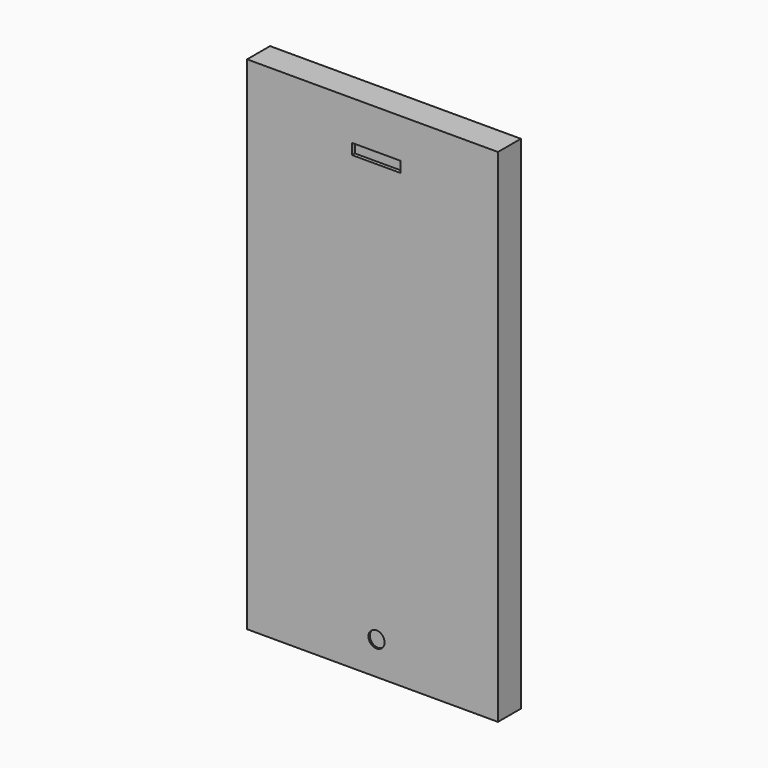
from build123d import *

# Parameters (mm, degrees)
F0_W     = 70
F0_H     = 140
F1_DEPTH = 8
F2_W     = 13.5
F2_H     = 3
F3_DEPTH = 1
F4_R     = 2.25
F5_DEPTH = 0.5
F6_R     = 5
F7_DEPTH = 1


# Not quite as in the source:
# - a feature of the source that left no trace in its solid (it failed there, or was rolled back) is left out


with BuildPart() as f1:
    # F0 (on Front) → F1 (new body)
    with BuildSketch(Plane.XZ):
        with Locations((5.7291688025, 19.6874958277)):
            Rectangle(F0_W, F0_H)
    extrude(amount=F1_DEPTH)

    # F2 (on face) → F3 (cut)
    with BuildSketch(Plane.XZ.offset(8)):
        with Locations((6.75, 77.1874958277)):
            Rectangle(F2_W, F2_H)
    extrude(amount=-F3_DEPTH, mode=Mode.SUBTRACT)

    # F4 (on face) → F5 (cut)
    with BuildSketch(Plane.XZ.offset(8)):
        with Locations((6.8374876864, -41.0625041723)):
            Circle(F4_R)
    extrude(amount=-F5_DEPTH, mode=Mode.SUBTRACT)

    # F6 (on face) → F7 (join)
    with BuildSketch(Plane(origin=(0, 0, 0), x_dir=(-1, 0, 0), z_dir=(0, 1, 0))):
        with Locations((-28.1465931075, 77.1049201327)):
            Circle(F6_R)
    extrude(amount=F7_DEPTH)


solid = f1.part
